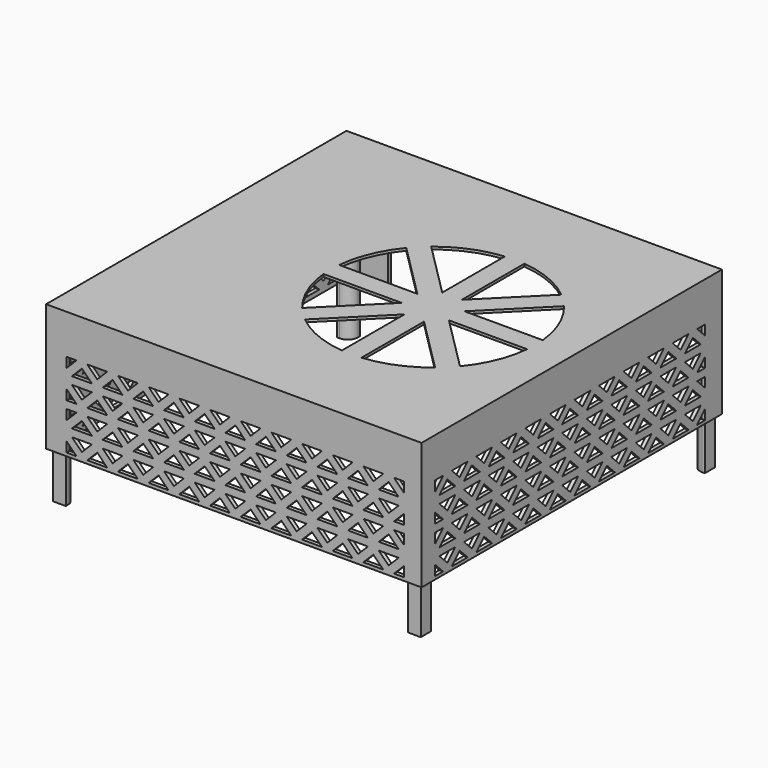
from build123d import *

# Parameters (mm, degrees)
F1_W      = 186.5100009048
F1_H      = 186.5100009048
F1_W_2    = 182.7000009048
F1_H_2    = 182.7000009048
F2_DEPTH  = 86.36
F5_W      = 186.5100009048
F5_H      = 186.5100009048
F6_DEPTH  = 1.27
F7_W      = 7.62
F7_H      = 7.62
F7_R      = 3.175
F7_R_2    = 1.27
F7_W_2    = 6.985
F7_H_2    = 33.02
F8_DEPTH  = 3.81
F9_R      = 1.27
F10_DEPTH = 6.35
F11_R     = 5.08
F11_R_2   = 5.3975
F11_R_3   = 3.175
F11_R_4   = 3.81
F12_DEPTH = 1.905
F13_W     = 10.668
F13_H     = 19.05
F14_DEPTH = 2.54
F15_W     = 16.51
F15_H     = 8.255
F15_R     = 1.905
F16_DEPTH = 1.905
F20_DEPTH = 0.9525
F21_R     = 1.27
F22_DEPTH = 12.7
F23_DEPTH = 25.4
F24_W     = 8.763
F24_H     = 45.085
F24_W_2   = 11.938
F24_W_3   = 10.16
F25_DEPTH = 25.4
F27_DEPTH = 1.905
F29_DEPTH = 2.54
F31_DEPTH = 2.54
F33_DEPTH = 2.54
F35_W     = 186.5100009048
F35_H     = 24.4348
F36_DEPTH = 186.5110009048
F37_W     = 159.385
F37_H     = 45.085
F38_DEPTH = 25.4
F39_W     = 182.7000009048
F39_H     = 182.7000009048
F40_DEPTH = 63.1962
F41_W     = 6.35
F41_H     = 6.35
F42_DEPTH = 86.36
F43_W     = 182.7000009048
F43_H     = 182.7000009048
F44_DEPTH = 1.27
F45_R     = 5.08


with BuildPart() as f2:
    # F1 (on Top) → F2 (new body)
    with BuildSketch(Plane.XY):
        with Locations((78.65, -74.84)):
            Rectangle(F1_W, F1_H)
        with Locations((78.65, -74.84)):
            Rectangle(F1_W_2, F1_H_2, mode=Mode.SUBTRACT)
    extrude(amount=F2_DEPTH)

    # F5 (on Top) → F6 (join)
    with BuildSketch(Plane.XY):
        with Locations((78.65, -74.84)):
            Rectangle(F5_W, F5_H)
    extrude(amount=-F6_DEPTH)

    # F7 (on Top) → F8 (join)
    with BuildSketch(Plane.XY):
        with Locations((81.7350004524, -95.2499995476)):
            Rectangle(F7_W, F7_H)
        with Locations((132.5350004524, -95.2499995476)):
            Rectangle(F7_W, F7_H)
        with Locations((83.0050004524, -5.0799995476)):
            Circle(F7_R)
        with Locations((83.0050004524, -5.0799995476)):
            Circle(F7_R_2, mode=Mode.SUBTRACT)
        with Locations((131.2650004524, 10.1600004524)):
            Circle(F7_R)
        with Locations((131.2650004524, 10.1600004524)):
            Circle(F7_R_2, mode=Mode.SUBTRACT)
        with Locations((50.9375004524, -41.2749995476)):
            Rectangle(F7_W_2, F7_H_2)
        with Locations((51.8900004524, -53.3399995476)):
            Circle(F7_R_2, mode=Mode.SUBTRACT)
        with Locations((51.8900004524, -26.6699995476)):
            Circle(F7_R_2, mode=Mode.SUBTRACT)
    extrude(amount=F8_DEPTH)

    # F9 (on Top) → F10 (join)
    with BuildSketch(Plane.XY):
        Polygon((76.0200004524, -15.2399995476), (67.8920004524, -15.2399995476), (67.8920004524, -24.7649995476), (69.7970004524, -24.7649995476), (69.7970004524, -17.1449995476), (77.9250004524, -17.1449995476), (77.9250004524, -1.2699995476), (69.7970004524, -1.2699995476), (69.7970004524, 16.5100004524), (67.8920004524, 16.5100004524), (67.8920004524, -3.1749995476), (76.0200004524, -3.1749995476), align=None)
        with BuildLine():
            Line((136.3450004524, 16.5100004524), (136.3450004524, -99.0599995476))
            Line((136.3450004524, -99.0599995476), (77.9250004524, -99.0599995476))
            Line((77.9250004524, -99.0599995476), (77.9250004524, -52.7049995476))
            Line((77.9250004524, -52.7049995476), (67.8920004524, -52.7049995476))
            Line((67.8920004524, -52.7049995476), (67.8920004524, -57.7849995476))
            Line((67.8920004524, -57.7849995476), (76.0200004524, -57.7849995476))
            Line((76.0200004524, -57.7849995476), (76.0200004524, -100.9649995476))
            Line((76.0200004524, -100.9649995476), (76.0200004524, -159.84))
            Line((76.0200004524, -159.84), (71.3210004524, -159.84))
            Line((71.3210004524, -159.84), (71.3210004524, -162.38))
            Line((71.3210004524, -162.38), (78.5600004524, -162.38))
            Line((78.5600004524, -162.38), (78.5600004524, -112.215))
            Line((78.5600004524, -112.215), (81.7350004524, -112.215))
            ThreePointArc((81.7350004524, -112.215), (84.9100004524, -109.04), (81.7350004524, -105.865))
            Line((81.7350004524, -105.865), (78.5600004524, -105.865))
            Line((78.5600004524, -105.865), (78.5600004524, -100.9649995476))
            Line((78.5600004524, -100.9649995476), (138.2500004524, -100.9649995476))
            Line((138.2500004524, -100.9649995476), (138.2500004524, 16.5100004524))
            Line((138.2500004524, 16.5100004524), (136.3450004524, 16.5100004524))
        make_face()
        with Locations((81.7350004524, -109.04)):
            Circle(F9_R, mode=Mode.SUBTRACT)
        with BuildLine():
            Line((5.6620004524, -57.7849995476), (47.4450004524, -57.7849995476))
            Line((47.4450004524, -57.7849995476), (47.4450004524, -55.2449995476))
            Line((47.4450004524, -55.2449995476), (3.1220004524, -55.2449995476))
            Line((3.1220004524, -55.2449995476), (3.1220004524, -105.865))
            Line((3.1220004524, -105.865), (-0.0529995476, -105.865))
            ThreePointArc((-0.0529995476, -105.865), (-3.2279995476, -109.04), (-0.0529995476, -112.215))
            Line((-0.0529995476, -112.215), (3.1220004524, -112.215))
            Line((3.1220004524, -112.215), (3.1220004524, -162.38))
            Line((3.1220004524, -162.38), (10.3610004524, -162.38))
            Line((10.3610004524, -162.38), (10.3610004524, -159.84))
            Line((10.3610004524, -159.84), (5.6620004524, -159.84))
            Line((5.6620004524, -159.84), (5.6620004524, -57.7849995476))
        make_face()
        with Locations((-0.0529995476, -109.04)):
            Circle(F9_R, mode=Mode.SUBTRACT)
    extrude(amount=F10_DEPTH)

    # F11 (on face) → F12 (cut, through all)
    with BuildSketch(Plane(origin=(0, 18.4150004524, 0), x_dir=(-1, 0, 0), z_dir=(0, 1, 0))):
        with Locations((-119.2000004524, 12.319)):
            Circle(F11_R)
        with Locations((-102.5630004524, 11.43)):
            Circle(F11_R_2)
        with Locations((-88.0850004524, 12.319)):
            Circle(F11_R_3)
        with Locations((-75.8930004524, 10.414)):
            Circle(F11_R_4)
    extrude(amount=-F12_DEPTH, mode=Mode.SUBTRACT)

    # F13 (on face) → F14 (cut)
    with BuildSketch(Plane(origin=(0, -166.1900004524, 0), x_dir=(-1, 0, 0), z_dir=(0, 1, 0))):
        Polygon((-10.3610004524, 0), (-10.3610004524, 6.35), (-10.3610004524, 19.05), (-16.7110004524, 19.05), (-16.7110004524, 0), align=None)
        with Locations((-22.8070004524, 9.525)):
            Rectangle(F13_W, F13_H)
        with Locations((-34.2370004524, 9.525)):
            Rectangle(F13_W, F13_H)
        with Locations((-45.6670004524, 9.525)):
            Rectangle(F13_W, F13_H)
        with Locations((-57.0970004524, 9.525)):
            Rectangle(F13_W, F13_H)
        Polygon((-71.3210004524, 6.35), (-71.3210004524, 0), (-63.1930004524, 0), (-63.1930004524, 19.05), (-71.3210004524, 19.05), align=None)
    extrude(amount=-F14_DEPTH, mode=Mode.SUBTRACT)

    # F15 (on face) → F16 (cut, through all)
    with BuildSketch(Plane.YZ.offset(171.9050004524)):
        with Locations((-125.73, 15.24)):
            Rectangle(F15_W, F15_H)
        with Locations((-141.605, 15.24)):
            Circle(F15_R)
        with Locations((-97.79, 15.24)):
            Rectangle(F15_W, F15_H)
        with Locations((-81.915, 15.24)):
            Circle(F15_R)
        with Locations((-54.61, 15.24)):
            Rectangle(F15_W, F15_H)
        with Locations((-69.215, 15.24)):
            Circle(F15_R)
        with Locations((-40.005, 15.24)):
            Circle(F15_R)
    extrude(amount=-F16_DEPTH, mode=Mode.SUBTRACT)

    # F19 (on plane+point) → F20 (join, symmetric)
    with BuildSketch(Plane.XZ.offset(75.565)):
        Polygon((170.0000004524, 0), (170.0000004524, 21.59), (157.3000004524, 0), align=None)
    extrude(amount=F20_DEPTH, both=True)

    # F21 (on Top) → F22 (join)
    with BuildSketch(Plane.XY):
        with BuildLine():
            ThreePointArc((-1.27, 2.9099355663), (0, 3.175), (1.27, 2.9099355663))
            Line((1.27, 2.9099355663), (1.27, 16.5100004524))
            Line((1.27, 16.5100004524), (-1.27, 16.5100004524))
            Line((-1.27, 16.5100004524), (-1.27, 2.9099355663))
        make_face()
        with BuildLine():
            Line((-12.7000004524, -1.27), (-2.9099355663, -1.27))
            ThreePointArc((-2.9099355663, -1.27), (-3.175, 0), (-2.9099355663, 1.27))
            Line((-2.9099355663, 1.27), (-12.7000004524, 1.27))
            Line((-12.7000004524, 1.27), (-12.7000004524, -1.27))
        make_face()
        Circle(F21_R)
        with Locations((157.48, -22.86)):
            Circle(F21_R)
        with BuildLine():
            ThreePointArc((160.3899355663, -21.59), (160.5880275436, -22.2113168813), (160.655, -22.86))
            ThreePointArc((160.655, -22.86), (160.5880275436, -23.5086831187), (160.3899355663, -24.13))
            Line((160.3899355663, -24.13), (170.0000004524, -24.13))
            Line((170.0000004524, -24.13), (170.0000004524, -21.59))
            Line((170.0000004524, -21.59), (160.3899355663, -21.59))
        make_face()
        with Locations((157.48, -154.94)):
            Circle(F21_R)
        with BuildLine():
            ThreePointArc((160.3899355663, -153.67), (160.5880275436, -154.2913168813), (160.655, -154.94))
            ThreePointArc((160.655, -154.94), (160.5880275436, -155.5886831187), (160.3899355663, -156.21))
            Line((160.3899355663, -156.21), (170.0000004524, -156.21))
            Line((170.0000004524, -156.21), (170.0000004524, -153.67))
            Line((170.0000004524, -153.67), (160.3899355663, -153.67))
        make_face()
        with BuildLine():
            ThreePointArc((158.75, -157.8499355663), (157.48, -158.115), (156.21, -157.8499355663))
            Line((156.21, -157.8499355663), (156.21, -166.1900004524))
            Line((156.21, -166.1900004524), (158.75, -166.1900004524))
            Line((158.75, -166.1900004524), (158.75, -157.8499355663))
        make_face()
        with BuildLine():
            ThreePointArc((-2.9099355663, -156.21), (-3.175, -154.94), (-2.9099355663, -153.67))
            Line((-2.9099355663, -153.67), (-12.7000004524, -153.67))
            Line((-12.7000004524, -153.67), (-12.7000004524, -156.21))
            Line((-12.7000004524, -156.21), (-2.9099355663, -156.21))
        make_face()
        with Locations((0, -154.94)):
            Circle(F21_R)
        with BuildLine():
            Line((1.27, -166.1900004524), (1.27, -157.8499355663))
            ThreePointArc((1.27, -157.8499355663), (0, -158.115), (-1.27, -157.8499355663))
            Line((-1.27, -157.8499355663), (-1.27, -166.1900004524))
            Line((-1.27, -166.1900004524), (1.27, -166.1900004524))
        make_face()
    extrude(amount=F22_DEPTH)

    # F21 (on Top) → F23 (join)
    with BuildSketch(Plane.XY):
        with BuildLine():
            ThreePointArc((-2.9099355663, -1.27), (0.6486831187, -3.1080275436), (3.175, 0))
            ThreePointArc((3.175, 0), (2.6563955842, 1.7390191201), (1.27, 2.9099355663))
            ThreePointArc((1.27, 2.9099355663), (0, 3.175), (-1.27, 2.9099355663))
            ThreePointArc((-1.27, 2.9099355663), (-2.2450640303, 2.2450640303), (-2.9099355663, 1.27))
            ThreePointArc((-2.9099355663, 1.27), (-3.175, 0), (-2.9099355663, -1.27))
        make_face()
        Circle(F21_R, mode=Mode.SUBTRACT)
        with BuildLine():
            ThreePointArc((160.3899355663, -24.13), (160.5880275436, -23.5086831187), (160.655, -22.86))
            ThreePointArc((160.655, -22.86), (160.5880275436, -22.2113168813), (160.3899355663, -21.59))
            ThreePointArc((160.3899355663, -21.59), (154.305, -22.86), (160.3899355663, -24.13))
        make_face()
        with Locations((157.48, -22.86)):
            Circle(F21_R, mode=Mode.SUBTRACT)
        with BuildLine():
            ThreePointArc((1.27, -157.8499355663), (2.6563955842, -156.6790191201), (3.175, -154.94))
            ThreePointArc((3.175, -154.94), (0.6486831187, -151.8319724564), (-2.9099355663, -153.67))
            ThreePointArc((-2.9099355663, -153.67), (-3.175, -154.94), (-2.9099355663, -156.21))
            ThreePointArc((-2.9099355663, -156.21), (-2.2450640303, -157.1850640303), (-1.27, -157.8499355663))
            ThreePointArc((-1.27, -157.8499355663), (0, -158.115), (1.27, -157.8499355663))
        make_face()
        with Locations((0, -154.94)):
            Circle(F21_R, mode=Mode.SUBTRACT)
        with BuildLine():
            ThreePointArc((160.3899355663, -156.21), (160.5880275436, -155.5886831187), (160.655, -154.94))
            ThreePointArc((160.655, -154.94), (160.5880275436, -154.2913168813), (160.3899355663, -153.67))
            ThreePointArc((160.3899355663, -153.67), (155.2349359697, -152.6949359697), (156.21, -157.8499355663))
            ThreePointArc((156.21, -157.8499355663), (157.48, -158.115), (158.75, -157.8499355663))
            ThreePointArc((158.75, -157.8499355663), (159.7250640303, -157.1850640303), (160.3899355663, -156.21))
        make_face()
        with Locations((157.48, -154.94)):
            Circle(F21_R, mode=Mode.SUBTRACT)
    extrude(amount=F23_DEPTH)

    # F24 (on Front) → F25 (cut)
    with BuildSketch(Plane.XZ):
        with Locations((11.8999, 45.7073)):
            Rectangle(F24_W, F24_H)
        with Locations((23.0124, 45.7073)):
            Rectangle(F24_W_2, F24_H)
        with Locations((35.7124, 45.7073)):
            Rectangle(F24_W_2, F24_H)
        with Locations((48.4124, 45.7073)):
            Rectangle(F24_W_2, F24_H)
        with Locations((61.1124, 45.7073)):
            Rectangle(F24_W_2, F24_H)
        with Locations((73.8124, 45.7073)):
            Rectangle(F24_W_2, F24_H)
        with Locations((86.5124, 45.7073)):
            Rectangle(F24_W_2, F24_H)
        with Locations((99.2124, 45.7073)):
            Rectangle(F24_W_2, F24_H)
        with Locations((111.9124, 45.7073)):
            Rectangle(F24_W_2, F24_H)
        with Locations((124.6124, 45.7073)):
            Rectangle(F24_W_2, F24_H)
        with Locations((137.3124, 45.7073)):
            Rectangle(F24_W_2, F24_H)
        with Locations((150.0124, 45.7073)):
            Rectangle(F24_W_2, F24_H)
        with Locations((161.8234, 45.7073)):
            Rectangle(F24_W_3, F24_H)
    extrude(amount=-F25_DEPTH, mode=Mode.SUBTRACT)

    # F26 (on face) → F27 (cut, through all)
    with BuildSketch(Plane.XZ.offset(-16.5100004524)):
        Polygon((23.3409231637, 9.525), (18.415, 9.525), (13.4890768363, 9.525), (18.415, 4.5990768363), align=None)
        Polygon((15.7209231637, 1.905), (10.795, 6.8309231637), (5.8690768363, 1.905), align=None)
        Polygon((3.175, 9.525), (3.175, 4.5990768363), (8.1009231637, 9.525), align=None)
        Polygon((33.655, 9.525), (28.7290768363, 9.525), (33.655, 4.5990768363), (38.5809231637, 9.525), align=None)
        Polygon((21.1090768363, 1.905), (30.9609231637, 1.905), (26.035, 6.8309231637), align=None)
        Polygon((41.275, 6.8309231637), (36.3490768363, 1.905), (46.2009231637, 1.905), align=None)
        Polygon((48.895, 9.525), (43.9690768363, 9.525), (48.895, 4.5990768363), (53.8209231637, 9.525), align=None)
        Polygon((8.1009231637, 13.335), (3.175, 18.2609231637), (3.175, 13.335), align=None)
        Polygon((15.7209231637, 20.955), (5.8690768363, 20.955), (10.795, 16.0290768363), align=None)
        Polygon((18.415, 18.2609231637), (13.4890768363, 13.335), (18.415, 13.335), (23.3409231637, 13.335), align=None)
        Polygon((21.1090768363, 20.955), (26.035, 16.0290768363), (30.9609231637, 20.955), align=None)
        Polygon((38.5809231637, 13.335), (33.655, 18.2609231637), (28.7290768363, 13.335), (33.655, 13.335), align=None)
        Polygon((36.3490768363, 20.955), (41.275, 16.0290768363), (46.2009231637, 20.955), align=None)
        Polygon((48.895, 18.2609231637), (43.9690768363, 13.335), (48.895, 13.335), (53.8209231637, 13.335), align=None)
        Polygon((51.5890768363, 20.955), (56.515, 16.0290768363), (61.4409231637, 20.955), align=None)
        Polygon((64.135, 13.335), (64.135, 18.2609231637), (59.2090768363, 13.335), align=None)
        Polygon((64.135, 9.525), (59.2090768363, 9.525), (64.135, 4.5990768363), align=None)
        Polygon((61.4409231637, 1.905), (56.515, 6.8309231637), (51.5890768363, 1.905), align=None)
        Polygon((138.2500004524, 9.525), (138.2500004524, 4.5990768363), (143.1759236161, 9.525), align=None)
        Polygon((140.9440772887, 20.955), (145.8700004524, 16.0290768363), (150.7959236161, 20.955), align=None)
        Polygon((143.1759236161, 13.335), (138.2500004524, 18.2609231637), (138.2500004524, 13.335), align=None)
        Polygon((168.7300004524, 13.335), (168.7300004524, 18.2609231637), (163.8040772887, 13.335), align=None)
        Polygon((158.4159236161, 9.525), (153.4900004524, 9.525), (148.5640772887, 9.525), (153.4900004524, 4.5990768363), align=None)
        Polygon((148.5640772887, 13.335), (153.4900004524, 13.335), (158.4159236161, 13.335), (153.4900004524, 18.2609231637), align=None)
        Polygon((168.7300004524, 9.525), (163.8040772887, 9.525), (168.7300004524, 4.5990768363), align=None)
        Polygon((161.1100004524, 20.955), (161.1100004524, 16.0290768363), (166.0359236161, 20.955), align=None)
        Polygon((156.1840772887, 20.955), (161.1100004524, 16.0290768363), (161.1100004524, 20.955), align=None)
        Polygon((161.1100004524, 1.905), (161.1100004524, 6.8309231637), (156.1840772887, 1.905), align=None)
        Polygon((166.0359236161, 1.905), (161.1100004524, 6.8309231637), (161.1100004524, 1.905), align=None)
        Polygon((150.7959236161, 1.905), (145.8700004524, 6.8309231637), (140.9440772887, 1.905), align=None)
    extrude(amount=-F27_DEPTH, mode=Mode.SUBTRACT)

    # F28 (on face) → F29 (cut)
    with BuildSketch(Plane.XZ.offset(168.0950004524)):
        Polygon((8.1009231637, 13.335), (3.175, 18.2609231637), (-1.7509231637, 13.335), (3.175, 13.335), align=None)
        Polygon((-4.445, 16.0290768363), (0.4809231637, 20.955), (-4.445, 20.955), align=None)
        Polygon((8.1009231637, 36.195), (3.175, 41.1209231637), (-1.7509231637, 36.195), (3.175, 36.195), align=None)
        Polygon((3.175, 32.385), (-1.7509231637, 32.385), (3.175, 27.4590768363), (8.1009231637, 32.385), align=None)
        Polygon((10.795, 29.6909231637), (5.8690768363, 24.765), (15.7209231637, 24.765), align=None)
        Polygon((15.7209231637, 43.815), (5.8690768363, 43.815), (10.795, 38.8890768363), align=None)
        Polygon((8.1009231637, 59.055), (3.175, 63.9809231637), (-1.7509231637, 59.055), (3.175, 59.055), align=None)
        Polygon((3.175, 55.245), (-1.7509231637, 55.245), (3.175, 50.3190768363), (8.1009231637, 55.245), align=None)
        Polygon((10.795, 52.5509231637), (5.8690768363, 47.625), (15.7209231637, 47.625), align=None)
        Polygon((15.7209231637, 66.675), (5.8690768363, 66.675), (10.795, 61.7490768363), align=None)
        Polygon((23.3409231637, 36.195), (18.415, 41.1209231637), (13.4890768363, 36.195), (18.415, 36.195), align=None)
        Polygon((18.415, 32.385), (13.4890768363, 32.385), (18.415, 27.4590768363), (23.3409231637, 32.385), align=None)
        Polygon((26.035, 29.6909231637), (21.1090768363, 24.765), (30.9609231637, 24.765), align=None)
        Polygon((30.9609231637, 43.815), (21.1090768363, 43.815), (26.035, 38.8890768363), align=None)
        Polygon((23.3409231637, 59.055), (18.415, 63.9809231637), (13.4890768363, 59.055), (18.415, 59.055), align=None)
        Polygon((18.415, 55.245), (13.4890768363, 55.245), (18.415, 50.3190768363), (23.3409231637, 55.245), align=None)
        Polygon((26.035, 52.5509231637), (21.1090768363, 47.625), (30.9609231637, 47.625), align=None)
        Polygon((30.9609231637, 66.675), (21.1090768363, 66.675), (26.035, 61.7490768363), align=None)
        Polygon((38.5809231637, 36.195), (33.655, 41.1209231637), (28.7290768363, 36.195), (33.655, 36.195), align=None)
        Polygon((33.655, 32.385), (28.7290768363, 32.385), (33.655, 27.4590768363), (38.5809231637, 32.385), align=None)
        Polygon((41.275, 29.6909231637), (36.3490768363, 24.765), (46.2009231637, 24.765), align=None)
        Polygon((46.2009231637, 43.815), (36.3490768363, 43.815), (41.275, 38.8890768363), align=None)
        Polygon((38.5809231637, 59.055), (33.655, 63.9809231637), (28.7290768363, 59.055), (33.655, 59.055), align=None)
        Polygon((33.655, 55.245), (28.7290768363, 55.245), (33.655, 50.3190768363), (38.5809231637, 55.245), align=None)
        Polygon((41.275, 52.5509231637), (36.3490768363, 47.625), (46.2009231637, 47.625), align=None)
        Polygon((46.2009231637, 66.675), (36.3490768363, 66.675), (41.275, 61.7490768363), align=None)
        Polygon((53.8209231637, 36.195), (48.895, 41.1209231637), (43.9690768363, 36.195), (48.895, 36.195), align=None)
        Polygon((48.895, 32.385), (43.9690768363, 32.385), (48.895, 27.4590768363), (53.8209231637, 32.385), align=None)
        Polygon((56.515, 29.6909231637), (51.5890768363, 24.765), (61.4409231637, 24.765), align=None)
        Polygon((61.4409231637, 43.815), (51.5890768363, 43.815), (56.515, 38.8890768363), align=None)
        Polygon((53.8209231637, 59.055), (48.895, 63.9809231637), (43.9690768363, 59.055), (48.895, 59.055), align=None)
        Polygon((48.895, 55.245), (43.9690768363, 55.245), (48.895, 50.3190768363), (53.8209231637, 55.245), align=None)
        Polygon((56.515, 52.5509231637), (51.5890768363, 47.625), (61.4409231637, 47.625), align=None)
        Polygon((61.4409231637, 66.675), (51.5890768363, 66.675), (56.515, 61.7490768363), align=None)
        Polygon((69.0609231637, 36.195), (64.135, 41.1209231637), (59.2090768363, 36.195), (64.135, 36.195), align=None)
        Polygon((64.135, 32.385), (59.2090768363, 32.385), (64.135, 27.4590768363), (69.0609231637, 32.385), align=None)
        Polygon((71.755, 29.6909231637), (66.8290768363, 24.765), (76.6809231637, 24.765), align=None)
        Polygon((76.6809231637, 43.815), (66.8290768363, 43.815), (71.755, 38.8890768363), align=None)
        Polygon((69.0609231637, 59.055), (64.135, 63.9809231637), (59.2090768363, 59.055), (64.135, 59.055), align=None)
        Polygon((64.135, 55.245), (59.2090768363, 55.245), (64.135, 50.3190768363), (69.0609231637, 55.245), align=None)
        Polygon((71.755, 52.5509231637), (66.8290768363, 47.625), (76.6809231637, 47.625), align=None)
        Polygon((76.6809231637, 66.675), (66.8290768363, 66.675), (71.755, 61.7490768363), align=None)
        Polygon((84.3009231637, 13.335), (79.375, 18.2609231637), (74.4490768363, 13.335), (79.375, 13.335), align=None)
        Polygon((79.375, 9.525), (74.4490768363, 9.525), (79.375, 4.5990768363), (84.3009231637, 9.525), align=None)
        Polygon((86.995, 6.8309231637), (82.0690768363, 1.905), (91.9209231637, 1.905), align=None)
        Polygon((91.9209231637, 20.955), (82.0690768363, 20.955), (86.995, 16.0290768363), align=None)
        Polygon((84.3009231637, 36.195), (79.375, 41.1209231637), (74.4490768363, 36.195), (79.375, 36.195), align=None)
        Polygon((79.375, 32.385), (74.4490768363, 32.385), (79.375, 27.4590768363), (84.3009231637, 32.385), align=None)
        Polygon((86.995, 29.6909231637), (82.0690768363, 24.765), (91.9209231637, 24.765), align=None)
        Polygon((91.9209231637, 43.815), (82.0690768363, 43.815), (86.995, 38.8890768363), align=None)
        Polygon((84.3009231637, 59.055), (79.375, 63.9809231637), (74.4490768363, 59.055), (79.375, 59.055), align=None)
        Polygon((79.375, 55.245), (74.4490768363, 55.245), (79.375, 50.3190768363), (84.3009231637, 55.245), align=None)
        Polygon((86.995, 52.5509231637), (82.0690768363, 47.625), (91.9209231637, 47.625), align=None)
        Polygon((91.9209231637, 66.675), (82.0690768363, 66.675), (86.995, 61.7490768363), align=None)
        Polygon((99.5409231637, 13.335), (94.615, 18.2609231637), (89.6890768363, 13.335), (94.615, 13.335), align=None)
        Polygon((94.615, 9.525), (89.6890768363, 9.525), (94.615, 4.5990768363), (99.5409231637, 9.525), align=None)
        Polygon((102.235, 6.8309231637), (97.3090768363, 1.905), (107.1609231637, 1.905), align=None)
        Polygon((107.1609231637, 20.955), (97.3090768363, 20.955), (102.235, 16.0290768363), align=None)
        Polygon((99.5409231637, 36.195), (94.615, 41.1209231637), (89.6890768363, 36.195), (94.615, 36.195), align=None)
        Polygon((94.615, 32.385), (89.6890768363, 32.385), (94.615, 27.4590768363), (99.5409231637, 32.385), align=None)
        Polygon((102.235, 29.6909231637), (97.3090768363, 24.765), (107.1609231637, 24.765), align=None)
        Polygon((107.1609231637, 43.815), (97.3090768363, 43.815), (102.235, 38.8890768363), align=None)
        Polygon((99.5409231637, 59.055), (94.615, 63.9809231637), (89.6890768363, 59.055), (94.615, 59.055), align=None)
        Polygon((94.615, 55.245), (89.6890768363, 55.245), (94.615, 50.3190768363), (99.5409231637, 55.245), align=None)
        Polygon((102.235, 52.5509231637), (97.3090768363, 47.625), (107.1609231637, 47.625), align=None)
        Polygon((107.1609231637, 66.675), (97.3090768363, 66.675), (102.235, 61.7490768363), align=None)
        Polygon((114.7809231637, 13.335), (109.855, 18.2609231637), (104.9290768363, 13.335), (109.855, 13.335), align=None)
        Polygon((109.855, 9.525), (104.9290768363, 9.525), (109.855, 4.5990768363), (114.7809231637, 9.525), align=None)
        Polygon((117.475, 6.8309231637), (112.5490768363, 1.905), (122.4009231637, 1.905), align=None)
        Polygon((122.4009231637, 20.955), (112.5490768363, 20.955), (117.475, 16.0290768363), align=None)
        Polygon((114.7809231637, 36.195), (109.855, 41.1209231637), (104.9290768363, 36.195), (109.855, 36.195), align=None)
        Polygon((109.855, 32.385), (104.9290768363, 32.385), (109.855, 27.4590768363), (114.7809231637, 32.385), align=None)
        Polygon((117.475, 29.6909231637), (112.5490768363, 24.765), (122.4009231637, 24.765), align=None)
        Polygon((122.4009231637, 43.815), (112.5490768363, 43.815), (117.475, 38.8890768363), align=None)
        Polygon((114.7809231637, 59.055), (109.855, 63.9809231637), (104.9290768363, 59.055), (109.855, 59.055), align=None)
        Polygon((109.855, 55.245), (104.9290768363, 55.245), (109.855, 50.3190768363), (114.7809231637, 55.245), align=None)
        Polygon((117.475, 52.5509231637), (112.5490768363, 47.625), (122.4009231637, 47.625), align=None)
        Polygon((122.4009231637, 66.675), (112.5490768363, 66.675), (117.475, 61.7490768363), align=None)
        Polygon((130.0209231637, 13.335), (125.095, 18.2609231637), (120.1690768363, 13.335), (125.095, 13.335), align=None)
        Polygon((125.095, 9.525), (120.1690768363, 9.525), (125.095, 4.5990768363), (130.0209231637, 9.525), align=None)
        Polygon((132.715, 6.8309231637), (127.7890768363, 1.905), (137.6409231637, 1.905), align=None)
        Polygon((137.6409231637, 20.955), (127.7890768363, 20.955), (132.715, 16.0290768363), align=None)
        Polygon((130.0209231637, 36.195), (125.095, 41.1209231637), (120.1690768363, 36.195), (125.095, 36.195), align=None)
        Polygon((125.095, 32.385), (120.1690768363, 32.385), (125.095, 27.4590768363), (130.0209231637, 32.385), align=None)
        Polygon((132.715, 29.6909231637), (127.7890768363, 24.765), (137.6409231637, 24.765), align=None)
        Polygon((137.6409231637, 43.815), (127.7890768363, 43.815), (132.715, 38.8890768363), align=None)
        Polygon((130.0209231637, 59.055), (125.095, 63.9809231637), (120.1690768363, 59.055), (125.095, 59.055), align=None)
        Polygon((125.095, 55.245), (120.1690768363, 55.245), (125.095, 50.3190768363), (130.0209231637, 55.245), align=None)
        Polygon((132.715, 52.5509231637), (127.7890768363, 47.625), (137.6409231637, 47.625), align=None)
        Polygon((137.6409231637, 66.675), (127.7890768363, 66.675), (132.715, 61.7490768363), align=None)
        Polygon((145.2609231637, 13.335), (140.335, 18.2609231637), (135.4090768363, 13.335), (140.335, 13.335), align=None)
        Polygon((140.335, 9.525), (135.4090768363, 9.525), (140.335, 4.5990768363), (145.2609231637, 9.525), align=None)
        Polygon((147.955, 6.8309231637), (143.0290768363, 1.905), (152.8809231637, 1.905), align=None)
        Polygon((152.8809231637, 20.955), (143.0290768363, 20.955), (147.955, 16.0290768363), align=None)
        Polygon((145.2609231637, 36.195), (140.335, 41.1209231637), (135.4090768363, 36.195), (140.335, 36.195), align=None)
        Polygon((140.335, 32.385), (135.4090768363, 32.385), (140.335, 27.4590768363), (145.2609231637, 32.385), align=None)
        Polygon((147.955, 29.6909231637), (143.0290768363, 24.765), (152.8809231637, 24.765), align=None)
        Polygon((152.8809231637, 43.815), (143.0290768363, 43.815), (147.955, 38.8890768363), align=None)
        Polygon((145.2609231637, 59.055), (140.335, 63.9809231637), (135.4090768363, 59.055), (140.335, 59.055), align=None)
        Polygon((140.335, 55.245), (135.4090768363, 55.245), (140.335, 50.3190768363), (145.2609231637, 55.245), align=None)
        Polygon((147.955, 52.5509231637), (143.0290768363, 47.625), (152.8809231637, 47.625), align=None)
        Polygon((152.8809231637, 66.675), (143.0290768363, 66.675), (147.955, 61.7490768363), align=None)
        Polygon((160.5009231637, 13.335), (155.575, 18.2609231637), (150.6490768363, 13.335), (155.575, 13.335), align=None)
        Polygon((163.195, 20.955), (158.2690768363, 20.955), (163.195, 16.0290768363), align=None)
        Polygon((160.5009231637, 36.195), (155.575, 41.1209231637), (150.6490768363, 36.195), (155.575, 36.195), align=None)
        Polygon((155.575, 32.385), (150.6490768363, 32.385), (155.575, 27.4590768363), (160.5009231637, 32.385), align=None)
        Polygon((163.195, 29.6909231637), (158.2690768363, 24.765), (163.195, 24.765), align=None)
        Polygon((163.195, 43.815), (158.2690768363, 43.815), (163.195, 38.8890768363), align=None)
        Polygon((160.5009231637, 59.055), (155.575, 63.9809231637), (150.6490768363, 59.055), (155.575, 59.055), align=None)
        Polygon((155.575, 55.245), (150.6490768363, 55.245), (155.575, 50.3190768363), (160.5009231637, 55.245), align=None)
        Polygon((163.195, 52.5509231637), (158.2690768363, 47.625), (163.195, 47.625), align=None)
        Polygon((163.195, 66.675), (158.2690768363, 66.675), (163.195, 61.7490768363), align=None)
        Polygon((-4.445, 43.815), (-4.445, 38.8890768363), (0.4809231637, 43.815), align=None)
        Polygon((0.4809231637, 24.765), (-4.445, 29.6909231637), (-4.445, 24.765), align=None)
        Polygon((-4.445, 66.675), (-4.445, 61.7490768363), (0.4809231637, 66.675), align=None)
        Polygon((0.4809231637, 47.625), (-4.445, 52.5509231637), (-4.445, 47.625), align=None)
    extrude(amount=-F29_DEPTH, mode=Mode.SUBTRACT)

    # F30 (on face) → F31 (cut)
    with BuildSketch(Plane.YZ.offset(171.9050004524)):
        Polygon((-147.1091767458, 58.98052284), (-152.0350999095, 63.9064460037), (-156.9610230731, 58.98052284), align=None)
        Polygon((-147.1091767458, 55.17052284), (-156.9610230731, 55.17052284), (-152.0350999095, 50.2445996763), align=None)
        Polygon((-144.4150999095, 52.4764460037), (-149.3410230731, 47.55052284), (-139.4891767458, 47.55052284), align=None)
        Polygon((-139.4891767458, 66.60052284), (-149.3410230731, 66.60052284), (-144.4150999095, 61.6745996763), align=None)
        Polygon((-131.8691767458, 58.98052284), (-136.7950999095, 63.9064460037), (-141.7210230731, 58.98052284), align=None)
        Polygon((-131.8691767458, 55.17052284), (-141.7210230731, 55.17052284), (-136.7950999095, 50.2445996763), align=None)
        Polygon((-129.1750999095, 52.4764460037), (-134.1010230731, 47.55052284), (-124.2491767458, 47.55052284), align=None)
        Polygon((-124.2491767458, 66.60052284), (-134.1010230731, 66.60052284), (-129.1750999095, 61.6745996763), align=None)
        Polygon((-116.6291767458, 58.98052284), (-121.5550999095, 63.9064460037), (-126.4810230731, 58.98052284), align=None)
        Polygon((-116.6291767458, 55.17052284), (-126.4810230731, 55.17052284), (-121.5550999095, 50.2445996763), align=None)
        Polygon((-113.9350999095, 52.4764460037), (-118.8610230731, 47.55052284), (-109.0091767458, 47.55052284), align=None)
        Polygon((-109.0091767458, 66.60052284), (-118.8610230731, 66.60052284), (-113.9350999095, 61.6745996763), align=None)
        Polygon((-101.3891767458, 58.98052284), (-106.3150999095, 63.9064460037), (-111.2410230731, 58.98052284), align=None)
        Polygon((-101.3891767458, 55.17052284), (-111.2410230731, 55.17052284), (-106.3150999095, 50.2445996763), align=None)
        Polygon((-98.6950999095, 52.4764460037), (-103.6210230731, 47.55052284), (-93.7691767458, 47.55052284), align=None)
        Polygon((-93.7691767458, 66.60052284), (-103.6210230731, 66.60052284), (-98.6950999095, 61.6745996763), align=None)
        Polygon((-86.1491767458, 58.98052284), (-91.0750999095, 63.9064460037), (-96.0010230731, 58.98052284), align=None)
        Polygon((-86.1491767458, 55.17052284), (-96.0010230731, 55.17052284), (-91.0750999095, 50.2445996763), align=None)
        Polygon((-83.4550999095, 52.4764460037), (-88.3810230731, 47.55052284), (-78.5291767458, 47.55052284), align=None)
        Polygon((-78.5291767458, 66.60052284), (-88.3810230731, 66.60052284), (-83.4550999095, 61.6745996763), align=None)
        Polygon((-70.9091767458, 58.98052284), (-75.8350999095, 63.9064460037), (-80.7610230731, 58.98052284), align=None)
        Polygon((-70.9091767458, 55.17052284), (-80.7610230731, 55.17052284), (-75.8350999095, 50.2445996763), align=None)
        Polygon((-68.2150999095, 52.4764460037), (-73.1410230731, 47.55052284), (-63.2891767458, 47.55052284), align=None)
        Polygon((-63.2891767458, 66.60052284), (-73.1410230731, 66.60052284), (-68.2150999095, 61.6745996763), align=None)
        Polygon((-55.6691767458, 58.98052284), (-60.5950999095, 63.9064460037), (-65.5210230731, 58.98052284), align=None)
        Polygon((-55.6691767458, 55.17052284), (-65.5210230731, 55.17052284), (-60.5950999095, 50.2445996763), align=None)
        Polygon((-52.9750999095, 52.4764460037), (-57.9010230731, 47.55052284), (-48.0491767458, 47.55052284), align=None)
        Polygon((-48.0491767458, 66.60052284), (-57.9010230731, 66.60052284), (-52.9750999095, 61.6745996763), align=None)
        Polygon((-40.4291767458, 58.98052284), (-45.3550999095, 63.9064460037), (-50.2810230731, 58.98052284), align=None)
        Polygon((-40.4291767458, 55.17052284), (-50.2810230731, 55.17052284), (-45.3550999095, 50.2445996763), align=None)
        Polygon((-37.7350999095, 52.4764460037), (-42.6610230731, 47.55052284), (-32.8091767458, 47.55052284), align=None)
        Polygon((-32.8091767458, 66.60052284), (-42.6610230731, 66.60052284), (-37.7350999095, 61.6745996763), align=None)
        Polygon((-25.1891767458, 58.98052284), (-30.1150999095, 63.9064460037), (-35.0410230731, 58.98052284), align=None)
        Polygon((-25.1891767458, 55.17052284), (-35.0410230731, 55.17052284), (-30.1150999095, 50.2445996763), align=None)
        Polygon((-22.4950999095, 52.4764460037), (-27.4210230731, 47.55052284), (-17.5691767458, 47.55052284), align=None)
        Polygon((-17.5691767458, 66.60052284), (-27.4210230731, 66.60052284), (-22.4950999095, 61.6745996763), align=None)
        Polygon((-9.9491767458, 58.98052284), (-14.8750999095, 63.9064460037), (-19.8010230731, 58.98052284), align=None)
        Polygon((-9.9491767458, 55.17052284), (-19.8010230731, 55.17052284), (-14.8750999095, 50.2445996763), align=None)
        Polygon((-7.2550999095, 52.4764460037), (-12.1810230731, 47.55052284), (-2.3291767458, 47.55052284), align=None)
        Polygon((-2.3291767458, 66.60052284), (-12.1810230731, 66.60052284), (-7.2550999095, 61.6745996763), align=None)
        Polygon((5.2908232542, 58.98052284), (0.3649000905, 63.9064460037), (-4.5610230731, 58.98052284), align=None)
        Polygon((5.2908232542, 55.17052284), (-4.5610230731, 55.17052284), (0.3649000905, 50.2445996763), align=None)
        Polygon((7.9849000905, 52.4764460037), (3.0589769269, 47.55052284), (7.9849000905, 47.55052284), align=None)
        Polygon((7.9849000905, 66.60052284), (3.0589769269, 66.60052284), (7.9849000905, 61.6745996763), align=None)
        Polygon((-159.6550999095, 66.60052284), (-159.6550999095, 61.6745996763), (-154.7291767458, 66.60052284), align=None)
        Polygon((-154.7291767458, 47.55052284), (-159.6550999095, 52.4764460037), (-159.6550999095, 47.55052284), align=None)
        Polygon((-121.5550999095, 41.0464460037), (-126.4810230731, 36.12052284), (-116.6291767458, 36.12052284), align=None)
        Polygon((-109.0091767458, 24.69052284), (-113.9350999095, 29.6164460037), (-118.8610230731, 24.69052284), align=None)
        Polygon((7.9849000905, 43.74052284), (3.0589769269, 43.74052284), (7.9849000905, 38.8145996763), align=None)
        Polygon((-126.4810230731, 32.31052284), (-121.5550999095, 27.3845996763), (-116.6291767458, 32.31052284), align=None)
        Polygon((-63.2891767458, 43.74052284), (-73.1410230731, 43.74052284), (-68.2150999095, 38.8145996763), align=None)
        Polygon((-98.6950999095, 29.6164460037), (-103.6210230731, 24.69052284), (-93.7691767458, 24.69052284), align=None)
        Polygon((-35.0410230731, 32.31052284), (-30.1150999095, 27.3845996763), (-25.1891767458, 32.31052284), align=None)
        Polygon((-32.8091767458, 43.74052284), (-42.6610230731, 43.74052284), (-37.7350999095, 38.8145996763), align=None)
        Polygon((-124.2491767458, 24.69052284), (-129.1750999095, 29.6164460037), (-134.1010230731, 24.69052284), align=None)
        Polygon((-4.5610230731, 32.31052284), (0.3649000905, 27.3845996763), (5.2908232542, 32.31052284), align=None)
        Polygon((-48.0491767458, 43.74052284), (-57.9010230731, 43.74052284), (-52.9750999095, 38.8145996763), align=None)
        Polygon((-19.8010230731, 32.31052284), (-14.8750999095, 27.3845996763), (-9.9491767458, 32.31052284), align=None)
        Polygon((-78.5291767458, 43.74052284), (-88.3810230731, 43.74052284), (-83.4550999095, 38.8145996763), align=None)
        Polygon((-101.3891767458, 36.12052284), (-106.3150999095, 41.0464460037), (-111.2410230731, 36.12052284), align=None)
        Polygon((-55.6691767458, 36.12052284), (-60.5950999095, 41.0464460037), (-65.5210230731, 36.12052284), align=None)
        Polygon((-152.0350999095, 41.0464460037), (-156.9610230731, 36.12052284), (-147.1091767458, 36.12052284), align=None)
        Polygon((-147.1091767458, 32.31052284), (-156.9610230731, 32.31052284), (-152.0350999095, 27.3845996763), align=None)
        Polygon((-139.4891767458, 24.69052284), (-144.4150999095, 29.6164460037), (-149.3410230731, 24.69052284), align=None)
        Polygon((-50.2810230731, 32.31052284), (-45.3550999095, 27.3845996763), (-40.4291767458, 32.31052284), align=None)
        Polygon((-124.2491767458, 43.74052284), (-134.1010230731, 43.74052284), (-129.1750999095, 38.8145996763), align=None)
        Polygon((-40.4291767458, 36.12052284), (-45.3550999095, 41.0464460037), (-50.2810230731, 36.12052284), align=None)
        Polygon((-111.2410230731, 32.31052284), (-106.3150999095, 27.3845996763), (-101.3891767458, 32.31052284), align=None)
        Polygon((-30.1150999095, 41.0464460037), (-35.0410230731, 36.12052284), (-25.1891767458, 36.12052284), align=None)
        Polygon((-27.4210230731, 43.74052284), (-22.4950999095, 38.8145996763), (-17.5691767458, 43.74052284), align=None)
        Polygon((-65.5210230731, 32.31052284), (-60.5950999095, 27.3845996763), (-55.6691767458, 32.31052284), align=None)
        Polygon((-14.8750999095, 41.0464460037), (-19.8010230731, 36.12052284), (-9.9491767458, 36.12052284), align=None)
        Polygon((-96.0010230731, 32.31052284), (-91.0750999095, 27.3845996763), (-86.1491767458, 32.31052284), align=None)
        Polygon((-93.7691767458, 43.74052284), (-103.6210230731, 43.74052284), (-98.6950999095, 38.8145996763), align=None)
        Polygon((-70.9091767458, 36.12052284), (-75.8350999095, 41.0464460037), (-80.7610230731, 36.12052284), align=None)
        Polygon((5.2908232542, 36.12052284), (0.3649000905, 41.0464460037), (-4.5610230731, 36.12052284), align=None)
        Polygon((-22.4950999095, 29.6164460037), (-27.4210230731, 24.69052284), (-17.5691767458, 24.69052284), align=None)
        Polygon((-48.0491767458, 24.69052284), (-52.9750999095, 29.6164460037), (-57.9010230731, 24.69052284), align=None)
        Polygon((-70.9091767458, 32.31052284), (-80.7610230731, 32.31052284), (-75.8350999095, 27.3845996763), align=None)
        Polygon((-7.2550999095, 29.6164460037), (-12.1810230731, 24.69052284), (-2.3291767458, 24.69052284), align=None)
        Polygon((-139.4891767458, 43.74052284), (-149.3410230731, 43.74052284), (-144.4150999095, 38.8145996763), align=None)
        Polygon((-2.3291767458, 43.74052284), (-12.1810230731, 43.74052284), (-7.2550999095, 38.8145996763), align=None)
        Polygon((-91.0750999095, 41.0464460037), (-96.0010230731, 36.12052284), (-86.1491767458, 36.12052284), align=None)
        Polygon((-37.7350999095, 29.6164460037), (-42.6610230731, 24.69052284), (-32.8091767458, 24.69052284), align=None)
        Polygon((-68.2150999095, 29.6164460037), (-73.1410230731, 24.69052284), (-63.2891767458, 24.69052284), align=None)
        Polygon((-78.5291767458, 24.69052284), (-83.4550999095, 29.6164460037), (-88.3810230731, 24.69052284), align=None)
        Polygon((7.9849000905, 29.6164460037), (3.0589769269, 24.69052284), (7.9849000905, 24.69052284), align=None)
        Polygon((-109.0091767458, 43.74052284), (-118.8610230731, 43.74052284), (-113.9350999095, 38.8145996763), align=None)
        Polygon((-131.8691767458, 36.12052284), (-136.7950999095, 41.0464460037), (-141.7210230731, 36.12052284), align=None)
        Polygon((-159.6550999095, 38.8145996763), (-154.7291767458, 43.74052284), (-159.6550999095, 43.74052284), align=None)
        Polygon((-131.8691767458, 32.31052284), (-141.7210230731, 32.31052284), (-136.7950999095, 27.3845996763), align=None)
        Polygon((-154.7291767458, 24.69052284), (-159.6550999095, 29.6164460037), (-159.6550999095, 24.69052284), align=None)
        Polygon((-109.0091767458, 1.83052284), (-113.9350999095, 6.7564460037), (-118.8610230731, 1.83052284), align=None)
        Polygon((7.9849000905, 20.88052284), (3.0589769269, 20.88052284), (7.9849000905, 15.9545996763), align=None)
        Polygon((-98.6950999095, 6.7564460037), (-103.6210230731, 1.83052284), (-93.7691767458, 1.83052284), align=None)
        Polygon((-124.2491767458, 1.83052284), (-129.1750999095, 6.7564460037), (-134.1010230731, 1.83052284), align=None)
        Polygon((-4.5610230731, 9.45052284), (0.3649000905, 4.5245996763), (5.2908232542, 9.45052284), align=None)
        Polygon((-14.8750999095, 9.45052284), (-14.8750999095, 4.5245996763), (-9.9491767458, 9.45052284), align=None)
        Polygon((-139.4891767458, 1.83052284), (-144.4150999095, 6.7564460037), (-149.3410230731, 1.83052284), align=None)
        Polygon((-14.8750999095, 18.1864460037), (-14.8750999095, 13.26052284), (-9.9491767458, 13.26052284), align=None)
        Polygon((5.2908232542, 13.26052284), (0.3649000905, 18.1864460037), (-4.5610230731, 13.26052284), align=None)
        Polygon((-48.0491767458, 1.83052284), (-52.9750999095, 6.7564460037), (-57.9010230731, 1.83052284), align=None)
        Polygon((-7.2550999095, 6.7564460037), (-12.1810230731, 1.83052284), (-2.3291767458, 1.83052284), align=None)
        Polygon((-2.3291767458, 20.88052284), (-12.1810230731, 20.88052284), (-7.2550999095, 15.9545996763), align=None)
        Polygon((-37.7350999095, 6.7564460037), (-42.6610230731, 1.83052284), (-32.8091767458, 1.83052284), align=None)
        Polygon((-68.2150999095, 6.7564460037), (-73.1410230731, 1.83052284), (-63.2891767458, 1.83052284), align=None)
        Polygon((-78.5291767458, 1.83052284), (-83.4550999095, 6.7564460037), (-88.3810230731, 1.83052284), align=None)
        Polygon((7.9849000905, 6.7564460037), (3.0589769269, 1.83052284), (7.9849000905, 1.83052284), align=None)
    extrude(amount=-F31_DEPTH, mode=Mode.SUBTRACT)

    # F32 (on face) → F33 (cut)
    with BuildSketch(Plane(origin=(-14.6050004524, 0, 0), x_dir=(0, -1, 0), z_dir=(-1, 0, 0))):
        Polygon((3.1267788771, 59.689999783), (-1.7991442865, 64.6159229467), (-6.7250674502, 59.689999783), align=None)
        Polygon((3.1267788771, 55.879999783), (-6.7250674502, 55.879999783), (-1.7991442865, 50.9540766194), align=None)
        Polygon((5.8208557135, 53.1859229467), (0.8949325498, 48.259999783), (10.7467788771, 48.259999783), align=None)
        Polygon((10.7467788771, 67.309999783), (0.8949325498, 67.309999783), (5.8208557135, 62.3840766194), align=None)
        Polygon((18.3667788771, 59.689999783), (13.4408557135, 64.6159229467), (8.5149325498, 59.689999783), align=None)
        Polygon((18.3667788771, 55.879999783), (8.5149325498, 55.879999783), (13.4408557135, 50.9540766194), align=None)
        Polygon((21.0608557135, 53.1859229467), (16.1349325498, 48.259999783), (25.9867788771, 48.259999783), align=None)
        Polygon((25.9867788771, 67.309999783), (16.1349325498, 67.309999783), (21.0608557135, 62.3840766194), align=None)
        Polygon((33.6067788771, 59.689999783), (28.6808557135, 64.6159229467), (23.7549325498, 59.689999783), align=None)
        Polygon((33.6067788771, 55.879999783), (23.7549325498, 55.879999783), (28.6808557135, 50.9540766194), align=None)
        Polygon((36.3008557135, 53.1859229467), (31.3749325498, 48.259999783), (41.2267788771, 48.259999783), align=None)
        Polygon((41.2267788771, 67.309999783), (31.3749325498, 67.309999783), (36.3008557135, 62.3840766194), align=None)
        Polygon((48.8467788771, 59.689999783), (43.9208557135, 64.6159229467), (38.9949325498, 59.689999783), align=None)
        Polygon((48.8467788771, 55.879999783), (38.9949325498, 55.879999783), (43.9208557135, 50.9540766194), align=None)
        Polygon((51.5408557135, 53.1859229467), (46.6149325498, 48.259999783), (56.4667788771, 48.259999783), align=None)
        Polygon((56.4667788771, 67.309999783), (46.6149325498, 67.309999783), (51.5408557135, 62.3840766194), align=None)
        Polygon((64.0867788771, 59.689999783), (59.1608557135, 64.6159229467), (54.2349325498, 59.689999783), align=None)
        Polygon((64.0867788771, 55.879999783), (54.2349325498, 55.879999783), (59.1608557135, 50.9540766194), align=None)
        Polygon((66.7808557135, 53.1859229467), (61.8549325498, 48.259999783), (71.7067788771, 48.259999783), align=None)
        Polygon((71.7067788771, 67.309999783), (61.8549325498, 67.309999783), (66.7808557135, 62.3840766194), align=None)
        Polygon((79.3267788771, 59.689999783), (74.4008557135, 64.6159229467), (69.4749325498, 59.689999783), align=None)
        Polygon((79.3267788771, 55.879999783), (69.4749325498, 55.879999783), (74.4008557135, 50.9540766194), align=None)
        Polygon((82.0208557135, 53.1859229467), (77.0949325498, 48.259999783), (86.9467788771, 48.259999783), align=None)
        Polygon((86.9467788771, 67.309999783), (77.0949325498, 67.309999783), (82.0208557135, 62.3840766194), align=None)
        Polygon((94.5667788771, 59.689999783), (89.6408557135, 64.6159229467), (84.7149325498, 59.689999783), align=None)
        Polygon((94.5667788771, 55.879999783), (84.7149325498, 55.879999783), (89.6408557135, 50.9540766194), align=None)
        Polygon((97.2608557135, 53.1859229467), (92.3349325498, 48.259999783), (102.1867788771, 48.259999783), align=None)
        Polygon((102.1867788771, 67.309999783), (92.3349325498, 67.309999783), (97.2608557135, 62.3840766194), align=None)
        Polygon((109.8067788771, 59.689999783), (104.8808557135, 64.6159229467), (99.9549325498, 59.689999783), align=None)
        Polygon((109.8067788771, 55.879999783), (99.9549325498, 55.879999783), (104.8808557135, 50.9540766194), align=None)
        Polygon((112.5008557135, 53.1859229467), (107.5749325498, 48.259999783), (117.4267788771, 48.259999783), align=None)
        Polygon((117.4267788771, 67.309999783), (107.5749325498, 67.309999783), (112.5008557135, 62.3840766194), align=None)
        Polygon((125.0467788771, 59.689999783), (120.1208557135, 64.6159229467), (115.1949325498, 59.689999783), align=None)
        Polygon((125.0467788771, 55.879999783), (115.1949325498, 55.879999783), (120.1208557135, 50.9540766194), align=None)
        Polygon((127.7408557135, 53.1859229467), (122.8149325498, 48.259999783), (132.6667788771, 48.259999783), align=None)
        Polygon((132.6667788771, 67.309999783), (122.8149325498, 67.309999783), (127.7408557135, 62.3840766194), align=None)
        Polygon((140.2867788771, 59.689999783), (135.3608557135, 64.6159229467), (130.4349325498, 59.689999783), align=None)
        Polygon((140.2867788771, 55.879999783), (130.4349325498, 55.879999783), (135.3608557135, 50.9540766194), align=None)
        Polygon((142.9808557135, 53.1859229467), (138.0549325498, 48.259999783), (147.9067788771, 48.259999783), align=None)
        Polygon((147.9067788771, 67.309999783), (138.0549325498, 67.309999783), (142.9808557135, 62.3840766194), align=None)
        Polygon((155.5267788771, 59.689999783), (150.6008557135, 64.6159229467), (145.6749325498, 59.689999783), align=None)
        Polygon((155.5267788771, 55.879999783), (145.6749325498, 55.879999783), (150.6008557135, 50.9540766194), align=None)
        Polygon((158.2208557135, 53.1859229467), (153.2949325498, 48.259999783), (158.2208557135, 48.259999783), align=None)
        Polygon((158.2208557135, 67.309999783), (153.2949325498, 67.309999783), (158.2208557135, 62.3840766194), align=None)
        Polygon((-9.4191442865, 67.309999783), (-9.4191442865, 62.3840766194), (-4.4932211229, 67.309999783), align=None)
        Polygon((-4.4932211229, 48.259999783), (-9.4191442865, 53.1859229467), (-9.4191442865, 48.259999783), align=None)
        Polygon((28.6808557135, 41.7559229467), (23.7549325498, 36.829999783), (33.6067788771, 36.829999783), align=None)
        Polygon((41.2267788771, 25.399999783), (36.3008557135, 30.3259229467), (31.3749325498, 25.399999783), align=None)
        Polygon((158.2208557135, 44.449999783), (153.2949325498, 44.449999783), (158.2208557135, 39.5240766194), align=None)
        Polygon((23.7549325498, 33.019999783), (28.6808557135, 28.0940766194), (33.6067788771, 33.019999783), align=None)
        Polygon((86.9467788771, 44.449999783), (77.0949325498, 44.449999783), (82.0208557135, 39.5240766194), align=None)
        Polygon((51.5408557135, 30.3259229467), (46.6149325498, 25.399999783), (56.4667788771, 25.399999783), align=None)
        Polygon((115.1949325498, 33.019999783), (120.1208557135, 28.0940766194), (125.0467788771, 33.019999783), align=None)
        Polygon((117.4267788771, 44.449999783), (107.5749325498, 44.449999783), (112.5008557135, 39.5240766194), align=None)
        Polygon((25.9867788771, 25.399999783), (21.0608557135, 30.3259229467), (16.1349325498, 25.399999783), align=None)
        Polygon((145.6749325498, 33.019999783), (150.6008557135, 28.0940766194), (155.5267788771, 33.019999783), align=None)
        Polygon((102.1867788771, 44.449999783), (92.3349325498, 44.449999783), (97.2608557135, 39.5240766194), align=None)
        Polygon((130.4349325498, 33.019999783), (135.3608557135, 28.0940766194), (140.2867788771, 33.019999783), align=None)
        Polygon((71.7067788771, 44.449999783), (61.8549325498, 44.449999783), (66.7808557135, 39.5240766194), align=None)
        Polygon((48.8467788771, 36.829999783), (43.9208557135, 41.7559229467), (38.9949325498, 36.829999783), align=None)
        Polygon((94.5667788771, 36.829999783), (89.6408557135, 41.7559229467), (84.7149325498, 36.829999783), align=None)
        Polygon((-1.7991442865, 41.7559229467), (-6.7250674502, 36.829999783), (3.1267788771, 36.829999783), align=None)
        Polygon((3.1267788771, 33.019999783), (-6.7250674502, 33.019999783), (-1.7991442865, 28.0940766194), align=None)
        Polygon((10.7467788771, 25.399999783), (5.8208557135, 30.3259229467), (0.8949325498, 25.399999783), align=None)
        Polygon((99.9549325498, 33.019999783), (104.8808557135, 28.0940766194), (109.8067788771, 33.019999783), align=None)
        Polygon((25.9867788771, 44.449999783), (16.1349325498, 44.449999783), (21.0608557135, 39.5240766194), align=None)
        Polygon((109.8067788771, 36.829999783), (104.8808557135, 41.7559229467), (99.9549325498, 36.829999783), align=None)
        Polygon((38.9949325498, 33.019999783), (43.9208557135, 28.0940766194), (48.8467788771, 33.019999783), align=None)
        Polygon((120.1208557135, 41.7559229467), (115.1949325498, 36.829999783), (125.0467788771, 36.829999783), align=None)
        Polygon((122.8149325498, 44.449999783), (127.7408557135, 39.5240766194), (132.6667788771, 44.449999783), align=None)
        Polygon((84.7149325498, 33.019999783), (89.6408557135, 28.0940766194), (94.5667788771, 33.019999783), align=None)
        Polygon((135.3608557135, 41.7559229467), (130.4349325498, 36.829999783), (140.2867788771, 36.829999783), align=None)
        Polygon((54.2349325498, 33.019999783), (59.1608557135, 28.0940766194), (64.0867788771, 33.019999783), align=None)
        Polygon((56.4667788771, 44.449999783), (46.6149325498, 44.449999783), (51.5408557135, 39.5240766194), align=None)
        Polygon((79.3267788771, 36.829999783), (74.4008557135, 41.7559229467), (69.4749325498, 36.829999783), align=None)
        Polygon((155.5267788771, 36.829999783), (150.6008557135, 41.7559229467), (145.6749325498, 36.829999783), align=None)
        Polygon((127.7408557135, 30.3259229467), (122.8149325498, 25.399999783), (132.6667788771, 25.399999783), align=None)
        Polygon((102.1867788771, 25.399999783), (97.2608557135, 30.3259229467), (92.3349325498, 25.399999783), align=None)
        Polygon((79.3267788771, 33.019999783), (69.4749325498, 33.019999783), (74.4008557135, 28.0940766194), align=None)
        Polygon((142.9808557135, 30.3259229467), (138.0549325498, 25.399999783), (147.9067788771, 25.399999783), align=None)
        Polygon((10.7467788771, 44.449999783), (0.8949325498, 44.449999783), (5.8208557135, 39.5240766194), align=None)
        Polygon((147.9067788771, 44.449999783), (138.0549325498, 44.449999783), (142.9808557135, 39.5240766194), align=None)
        Polygon((59.1608557135, 41.7559229467), (54.2349325498, 36.829999783), (64.0867788771, 36.829999783), align=None)
        Polygon((112.5008557135, 30.3259229467), (107.5749325498, 25.399999783), (117.4267788771, 25.399999783), align=None)
        Polygon((82.0208557135, 30.3259229467), (77.0949325498, 25.399999783), (86.9467788771, 25.399999783), align=None)
        Polygon((71.7067788771, 25.399999783), (66.7808557135, 30.3259229467), (61.8549325498, 25.399999783), align=None)
        Polygon((158.2208557135, 30.3259229467), (153.2949325498, 25.399999783), (158.2208557135, 25.399999783), align=None)
        Polygon((41.2267788771, 44.449999783), (31.3749325498, 44.449999783), (36.3008557135, 39.5240766194), align=None)
        Polygon((18.3667788771, 36.829999783), (13.4408557135, 41.7559229467), (8.5149325498, 36.829999783), align=None)
        Polygon((-9.4191442865, 39.5240766194), (-4.4932211229, 44.449999783), (-9.4191442865, 44.449999783), align=None)
        Polygon((18.3667788771, 33.019999783), (8.5149325498, 33.019999783), (13.4408557135, 28.0940766194), align=None)
        Polygon((-4.4932211229, 25.399999783), (-9.4191442865, 30.3259229467), (-9.4191442865, 25.399999783), align=None)
        Polygon((28.6808557135, 18.8959229467), (23.7549325498, 13.969999783), (33.6067788771, 13.969999783), align=None)
        Polygon((41.2267788771, 2.539999783), (36.3008557135, 7.4659229467), (31.3749325498, 2.539999783), align=None)
        Polygon((158.2208557135, 21.589999783), (153.2949325498, 21.589999783), (158.2208557135, 16.6640766194), align=None)
        Polygon((23.7549325498, 10.159999783), (28.6808557135, 5.2340766194), (33.6067788771, 10.159999783), align=None)
        Polygon((86.9467788771, 21.589999783), (77.0949325498, 21.589999783), (82.0208557135, 16.6640766194), align=None)
        Polygon((51.5408557135, 7.4659229467), (46.6149325498, 2.539999783), (56.4667788771, 2.539999783), align=None)
        Polygon((115.1949325498, 10.159999783), (120.1208557135, 5.2340766194), (125.0467788771, 10.159999783), align=None)
        Polygon((117.4267788771, 21.589999783), (107.5749325498, 21.589999783), (112.5008557135, 16.6640766194), align=None)
        Polygon((25.9867788771, 2.539999783), (21.0608557135, 7.4659229467), (16.1349325498, 2.539999783), align=None)
        Polygon((102.1867788771, 21.589999783), (92.3349325498, 21.589999783), (97.2608557135, 16.6640766194), align=None)
        Polygon((130.4349325498, 10.159999783), (135.3608557135, 5.2340766194), (140.2867788771, 10.159999783), align=None)
        Polygon((71.7067788771, 21.589999783), (61.8549325498, 21.589999783), (66.7808557135, 16.6640766194), align=None)
        Polygon((48.8467788771, 13.969999783), (43.9208557135, 18.8959229467), (38.9949325498, 13.969999783), align=None)
        Polygon((94.5667788771, 13.969999783), (89.6408557135, 18.8959229467), (84.7149325498, 13.969999783), align=None)
        Polygon((-1.7991442865, 18.8959229467), (-6.7250674502, 13.969999783), (3.1267788771, 13.969999783), align=None)
        Polygon((-1.7991442865, 10.159999783), (-6.7250674502, 10.159999783), (-1.7991442865, 5.2340766194), align=None)
        Polygon((10.7467788771, 2.539999783), (5.8208557135, 7.4659229467), (5.8208557135, 2.539999783), align=None)
        Polygon((99.9549325498, 10.159999783), (104.8808557135, 5.2340766194), (109.8067788771, 10.159999783), align=None)
        Polygon((25.9867788771, 21.589999783), (16.1349325498, 21.589999783), (21.0608557135, 16.6640766194), align=None)
        Polygon((109.8067788771, 13.969999783), (104.8808557135, 18.8959229467), (99.9549325498, 13.969999783), align=None)
        Polygon((145.6749325498, 10.159999783), (150.6008557135, 5.2340766194), (150.6008557135, 10.159999783), align=None)
        Polygon((38.9949325498, 10.159999783), (43.9208557135, 5.2340766194), (48.8467788771, 10.159999783), align=None)
        Polygon((120.1208557135, 18.8959229467), (115.1949325498, 13.969999783), (125.0467788771, 13.969999783), align=None)
        Polygon((122.8149325498, 21.589999783), (127.7408557135, 16.6640766194), (132.6667788771, 21.589999783), align=None)
        Polygon((84.7149325498, 10.159999783), (89.6408557135, 5.2340766194), (94.5667788771, 10.159999783), align=None)
        Polygon((135.3608557135, 18.8959229467), (130.4349325498, 13.969999783), (140.2867788771, 13.969999783), align=None)
        Polygon((54.2349325498, 10.159999783), (59.1608557135, 5.2340766194), (64.0867788771, 10.159999783), align=None)
        Polygon((56.4667788771, 21.589999783), (46.6149325498, 21.589999783), (51.5408557135, 16.6640766194), align=None)
        Polygon((79.3267788771, 13.969999783), (74.4008557135, 18.8959229467), (69.4749325498, 13.969999783), align=None)
        Polygon((155.5267788771, 13.969999783), (150.6008557135, 18.8959229467), (145.6749325498, 13.969999783), align=None)
        Polygon((127.7408557135, 7.4659229467), (122.8149325498, 2.539999783), (132.6667788771, 2.539999783), align=None)
        Polygon((102.1867788771, 2.539999783), (97.2608557135, 7.4659229467), (92.3349325498, 2.539999783), align=None)
        Polygon((79.3267788771, 10.159999783), (69.4749325498, 10.159999783), (74.4008557135, 5.2340766194), align=None)
        Polygon((142.9808557135, 7.4659229467), (138.0549325498, 2.539999783), (147.9067788771, 2.539999783), align=None)
        Polygon((10.7467788771, 21.589999783), (0.8949325498, 21.589999783), (5.8208557135, 16.6640766194), align=None)
        Polygon((147.9067788771, 21.589999783), (138.0549325498, 21.589999783), (142.9808557135, 16.6640766194), align=None)
        Polygon((59.1608557135, 18.8959229467), (54.2349325498, 13.969999783), (64.0867788771, 13.969999783), align=None)
        Polygon((112.5008557135, 7.4659229467), (107.5749325498, 2.539999783), (117.4267788771, 2.539999783), align=None)
        Polygon((82.0208557135, 7.4659229467), (77.0949325498, 2.539999783), (86.9467788771, 2.539999783), align=None)
        Polygon((71.7067788771, 2.539999783), (66.7808557135, 7.4659229467), (61.8549325498, 2.539999783), align=None)
        Polygon((41.2267788771, 21.589999783), (31.3749325498, 21.589999783), (36.3008557135, 16.6640766194), align=None)
        Polygon((18.3667788771, 13.969999783), (13.4408557135, 18.8959229467), (8.5149325498, 13.969999783), align=None)
        Polygon((-9.4191442865, 16.6640766194), (-4.4932211229, 21.589999783), (-9.4191442865, 21.589999783), align=None)
        Polygon((18.3667788771, 10.159999783), (8.5149325498, 10.159999783), (13.4408557135, 5.2340766194), align=None)
        Polygon((-4.4932211229, 2.539999783), (-9.4191442865, 7.4659229467), (-9.4191442865, 2.539999783), align=None)
    extrude(amount=-F33_DEPTH, mode=Mode.SUBTRACT)

    # F35 (on face) → F36 (cut, through all)
    with BuildSketch(Plane(origin=(0, 18.4150004524, 0), x_dir=(-1, 0, 0), z_dir=(0, 1, 0))):
        with Locations((-78.65, 10.9474)):
            Rectangle(F35_W, F35_H)
    extrude(amount=-F36_DEPTH, mode=Mode.SUBTRACT)

    # F37 (on face) → F38 (cut)
    with BuildSketch(Plane(origin=(0, 18.4150004524, 0), x_dir=(-1, 0, 0), z_dir=(0, 1, 0))):
        with Locations((-87.2109, 45.7073)):
            Rectangle(F37_W, F37_H)
    extrude(amount=-F38_DEPTH, mode=Mode.SUBTRACT)

    # F39 (on face) → F40 (cut, through all)
    with BuildSketch(Plane.XY.offset(86.36)):
        with Locations((78.65, -74.84)):
            Rectangle(F39_W, F39_H)
    extrude(amount=-F40_DEPTH, mode=Mode.SUBTRACT)

    # F41 (on face) → F42 (join, through all)
    with BuildSketch(Plane.XY.offset(86.36)):
        with Locations((-9.5250004524, 13.3350004524)):
            Rectangle(F41_W, F41_H)
        with Locations((166.8250004524, 13.3350004524)):
            Rectangle(F41_W, F41_H)
        with Locations((166.8250004524, -163.0150004524)):
            Rectangle(F41_W, F41_H)
        with Locations((-9.5250004524, -163.0150004524)):
            Rectangle(F41_W, F41_H)
    extrude(amount=-F42_DEPTH)

    # F43 (on offset) → F44 (join, through all)
    with BuildSketch(Plane.XY.offset(85.09)):
        with Locations((78.65, -74.84)):
            Rectangle(F43_W, F43_H)
        with BuildLine():
            Line((53.5730184175, -81.060079591), (92.4067299371, -81.060079591))
            Line((92.4067299371, -81.060079591), (64.9471491829, -108.5196603452))
            ThreePointArc((64.9471491829, -108.5196603452), (57.2069197484, -95.6403183641), (53.5730184175, -81.060079591))
        make_face(mode=Mode.SUBTRACT)
        with BuildLine():
            Line((71.8203396548, -115.3928508171), (99.279920409, -87.9332700629))
            Line((99.279920409, -87.9332700629), (99.279920409, -126.7669815825))
            ThreePointArc((99.279920409, -126.7669815825), (84.6996816359, -123.1330802516), (71.8203396548, -115.3928508171))
        make_face(mode=Mode.SUBTRACT)
        with BuildLine():
            Line((109.000079591, -126.7669815825), (109.000079591, -87.9332700629))
            Line((109.000079591, -87.9332700629), (136.4596603452, -115.3928508171))
            ThreePointArc((136.4596603452, -115.3928508171), (123.5803183641, -123.1330802516), (109.000079591, -126.7669815825))
        make_face(mode=Mode.SUBTRACT)
        with BuildLine():
            Line((143.3328508171, -108.5196603452), (115.8732700629, -81.060079591))
            Line((115.8732700629, -81.060079591), (154.7069815825, -81.060079591))
            ThreePointArc((154.7069815825, -81.060079591), (151.0730802516, -95.6403183641), (143.3328508171, -108.5196603452))
        make_face(mode=Mode.SUBTRACT)
        with BuildLine():
            Line((64.9471491829, -43.8803396548), (92.4067299371, -71.339920409))
            Line((92.4067299371, -71.339920409), (53.5730184175, -71.339920409))
            ThreePointArc((53.5730184175, -71.339920409), (57.2069197484, -56.7596816359), (64.9471491829, -43.8803396548))
        make_face(mode=Mode.SUBTRACT)
        with BuildLine():
            Line((99.279920409, -25.6330184175), (99.279920409, -64.4667299371))
            Line((99.279920409, -64.4667299371), (71.8203396548, -37.0071491829))
            ThreePointArc((71.8203396548, -37.0071491829), (84.6996816359, -29.2669197484), (99.279920409, -25.6330184175))
        make_face(mode=Mode.SUBTRACT)
        with BuildLine():
            Line((136.4596603452, -37.0071491829), (109.000079591, -64.4667299371))
            Line((109.000079591, -64.4667299371), (109.000079591, -25.6330184175))
            ThreePointArc((109.000079591, -25.6330184175), (123.5803183641, -29.2669197484), (136.4596603452, -37.0071491829))
        make_face(mode=Mode.SUBTRACT)
        with BuildLine():
            Line((154.7069815825, -71.339920409), (115.8732700629, -71.339920409))
            Line((115.8732700629, -71.339920409), (143.3328508171, -43.8803396548))
            ThreePointArc((143.3328508171, -43.8803396548), (151.0730802516, -56.7596816359), (154.7069815825, -71.339920409))
        make_face(mode=Mode.SUBTRACT)
    extrude(amount=F44_DEPTH)

    # F45
    f45_edges = [f2.edges().sort_by_distance(p)[0] for p in [
        (-6.35, -159.84, 42.545),
        (163.65, -159.84, 42.545),
        (163.65, 10.16, 42.545),
        (-6.35, 10.16, 42.545),
    ]]
    fillet(f45_edges, radius=F45_R)


solid = f2.part
